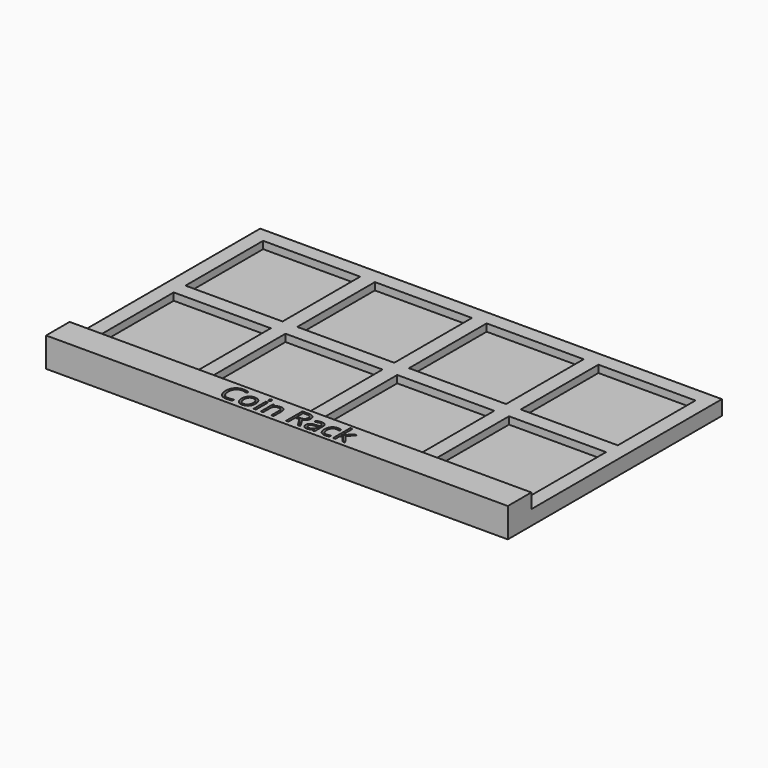
from build123d import *

# Parameters (mm, degrees)
F0_W         = 157
F0_H         = 81
F0_W_2       = 33
F0_H_2       = 33
F1_DEPTH     = 5
F2_DEPTH     = 2.5
F0_H_3       = 10
F3_DEPTH     = 10
F4_TEXT_SIZE = 9.7222222222
F5_DEPTH     = 2


# Not quite as in the source:
# - Text() gives the source's letters only with a copy of the font that has no kerning and outlines rounded to 1/6400 em; it was checked with that copy


with BuildPart() as f1:
    # F0 (on Top) → F1 (new body)
    with BuildSketch(Plane.XY):
        Rectangle(F0_W, F0_H)
        with Locations((-57, -19)):
            Rectangle(F0_W_2, F0_H_2, mode=Mode.SUBTRACT)
        with Locations((-19, -19)):
            Rectangle(F0_W_2, F0_H_2, mode=Mode.SUBTRACT)
        with Locations((19, -19)):
            Rectangle(F0_W_2, F0_H_2, mode=Mode.SUBTRACT)
        with Locations((57, -19)):
            Rectangle(F0_W_2, F0_H_2, mode=Mode.SUBTRACT)
        with Locations((-57, 19)):
            Rectangle(F0_W_2, F0_H_2, mode=Mode.SUBTRACT)
        with Locations((-19, 19)):
            Rectangle(F0_W_2, F0_H_2, mode=Mode.SUBTRACT)
        with Locations((19, 19)):
            Rectangle(F0_W_2, F0_H_2, mode=Mode.SUBTRACT)
        with Locations((57, 19)):
            Rectangle(F0_W_2, F0_H_2, mode=Mode.SUBTRACT)
    extrude(amount=F1_DEPTH)

    # F0 (on Top) → F2 (join)
    with BuildSketch(Plane.XY):
        with Locations((19, -19)):
            Rectangle(F0_W_2, F0_H_2)
        with Locations((57, -19)):
            Rectangle(F0_W_2, F0_H_2)
        with Locations((57, 19)):
            Rectangle(F0_W_2, F0_H_2)
        with Locations((19, 19)):
            Rectangle(F0_W_2, F0_H_2)
        with Locations((-19, 19)):
            Rectangle(F0_W_2, F0_H_2)
        with Locations((-57, 19)):
            Rectangle(F0_W_2, F0_H_2)
        with Locations((-57, -19)):
            Rectangle(F0_W_2, F0_H_2)
        with Locations((-19, -19)):
            Rectangle(F0_W_2, F0_H_2)
    extrude(amount=F2_DEPTH)

    # F0 (on Top) → F3 (join)
    with BuildSketch(Plane.XY):
        with Locations((0, -45.5)):
            Rectangle(F0_W, F0_H_3)
    extrude(amount=F3_DEPTH)

    # F4 (on face) → F5 (cut)
    with BuildSketch(Plane.XY.offset(10)):
        with Locations((-22.0018446181, -49)):
            Text('Coin Rack', F4_TEXT_SIZE, font='Open Sans', text_align=(TextAlign.LEFT, TextAlign.BOTTOM))
    extrude(amount=-F5_DEPTH, mode=Mode.SUBTRACT)


solid = f1.part
